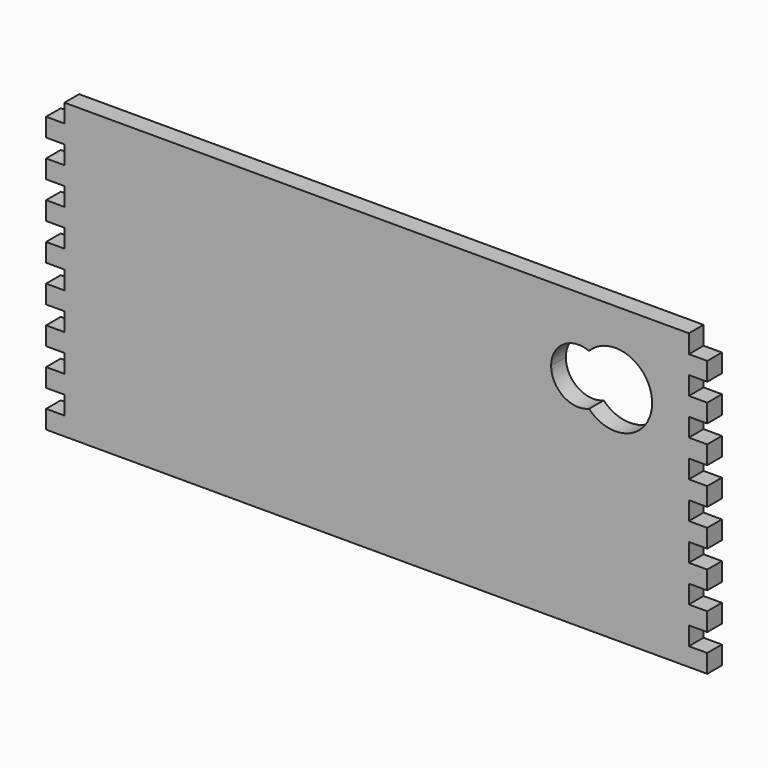
from build123d import *

# Parameters (mm, degrees)
F0_W     = 3.175
F0_H     = 3.175
F0_W_2   = 69.85
F0_H_2   = 12.7
F1_DEPTH = 3.175


with BuildPart() as f1:
    # F0 (on Front) → F1 (new body)
    with BuildSketch(Plane.XZ):
        Polygon((-67.174376142, 48.1953912664), (-79.874376142, 48.1953912664), (-79.874376142, 45.0203912664), (-79.874376142, 41.8453912664), (-79.874376142, 38.6703912664), (-79.874376142, 35.4953912664), (-67.174376142, 35.4953912664), align=None)
        with Locations((-81.461876142, 43.4328912664)):
            Rectangle(F0_W, F0_H)
        with Locations((-32.249376142, 41.8453912664)):
            Rectangle(F0_W_2, F0_H_2)
        with BuildLine():
            Line((15.375623858, 48.1953912664), (2.675623858, 48.1953912664))
            Line((2.675623858, 48.1953912664), (2.675623858, 35.4953912664))
            Line((2.675623858, 35.4953912664), (4.263123858, 35.4953912664))
            ThreePointArc((4.263123858, 35.4953912664), (6.3633054223, 39.4442476574), (10.811561358, 39.9103469283))
            ThreePointArc((10.811561358, 39.9103469283), (12.8969617645, 41.3416494053), (15.375623858, 41.8453912664))
            Line((15.375623858, 41.8453912664), (15.375623858, 48.1953912664))
        make_face()
        with BuildLine():
            Line((2.675623858, 35.4953912664), (-67.174376142, 35.4953912664))
            Line((-67.174376142, 35.4953912664), (-67.174376142, -2.6046087336))
            Line((-67.174376142, -2.6046087336), (28.075623858, -2.6046087336))
            Line((28.075623858, -2.6046087336), (28.075623858, 0.5703912664))
            Line((28.075623858, 0.5703912664), (28.075623858, 3.7453912664))
            Line((28.075623858, 3.7453912664), (28.075623858, 6.9203912664))
            Line((28.075623858, 6.9203912664), (28.075623858, 10.0953912664))
            Line((28.075623858, 10.0953912664), (28.075623858, 13.2703912664))
            Line((28.075623858, 13.2703912664), (28.075623858, 16.4453912664))
            Line((28.075623858, 16.4453912664), (28.075623858, 19.6203912664))
            Line((28.075623858, 19.6203912664), (28.075623858, 22.7953912664))
            Line((28.075623858, 22.7953912664), (28.075623858, 25.9703912664))
            Line((28.075623858, 25.9703912664), (28.075623858, 29.1453912664))
            Line((28.075623858, 29.1453912664), (28.075623858, 32.3203912664))
            Line((28.075623858, 32.3203912664), (28.075623858, 35.4953912664))
            Line((28.075623858, 35.4953912664), (21.725623858, 35.4953912664))
            ThreePointArc((21.725623858, 35.4953912664), (17.756873858, 29.6087837173), (10.811561358, 31.0804356046))
            ThreePointArc((10.811561358, 31.0804356046), (6.3633054223, 31.5465348754), (4.263123858, 35.4953912664))
            Line((4.263123858, 35.4953912664), (2.675623858, 35.4953912664))
        make_face()
        Polygon((-67.174376142, -2.6046087336), (-67.174376142, 35.4953912664), (-79.874376142, 35.4953912664), (-79.874376142, 32.3203912664), (-79.874376142, 29.1453912664), (-79.874376142, 25.9703912664), (-79.874376142, 22.7953912664), (-79.874376142, 19.6203912664), (-79.874376142, 16.4453912664), (-79.874376142, 13.2703912664), (-79.874376142, 10.0953912664), (-79.874376142, 6.9203912664), (-79.874376142, 3.7453912664), (-79.874376142, 0.5703912664), (-79.874376142, -2.6046087336), align=None)
        with Locations((-81.461876142, 37.0828912664)):
            Rectangle(F0_W, F0_H)
        with BuildLine():
            Line((28.075623858, 48.1953912664), (15.375623858, 48.1953912664))
            Line((15.375623858, 48.1953912664), (15.375623858, 41.8453912664))
            ThreePointArc((15.375623858, 41.8453912664), (19.8657519185, 39.985519327), (21.725623858, 35.4953912664))
            Line((21.725623858, 35.4953912664), (28.075623858, 35.4953912664))
            Line((28.075623858, 35.4953912664), (28.075623858, 38.6703912664))
            Line((28.075623858, 38.6703912664), (28.075623858, 41.8453912664))
            Line((28.075623858, 41.8453912664), (28.075623858, 45.0203912664))
            Line((28.075623858, 45.0203912664), (28.075623858, 48.1953912664))
        make_face()
        with Locations((-81.461876142, -1.0171087336)):
            Rectangle(F0_W, F0_H)
        with Locations((29.663123858, -1.0171087336)):
            Rectangle(F0_W, F0_H)
        with Locations((-81.461876142, 30.7328912664)):
            Rectangle(F0_W, F0_H)
        with Locations((29.663123858, 43.4328912664)):
            Rectangle(F0_W, F0_H)
        with Locations((29.663123858, 37.0828912664)):
            Rectangle(F0_W, F0_H)
        with Locations((-81.461876142, 5.3328912664)):
            Rectangle(F0_W, F0_H)
        with Locations((29.663123858, 5.3328912664)):
            Rectangle(F0_W, F0_H)
        with Locations((-81.461876142, 24.3828912664)):
            Rectangle(F0_W, F0_H)
        with Locations((29.663123858, 30.7328912664)):
            Rectangle(F0_W, F0_H)
        with Locations((-81.461876142, 11.6828912664)):
            Rectangle(F0_W, F0_H)
        with Locations((29.663123858, 11.6828912664)):
            Rectangle(F0_W, F0_H)
        with Locations((-81.461876142, 18.0328912664)):
            Rectangle(F0_W, F0_H)
        with Locations((29.663123858, 24.3828912664)):
            Rectangle(F0_W, F0_H)
        with Locations((29.663123858, 18.0328912664)):
            Rectangle(F0_W, F0_H)
    extrude(amount=F1_DEPTH)


solid = f1.part
